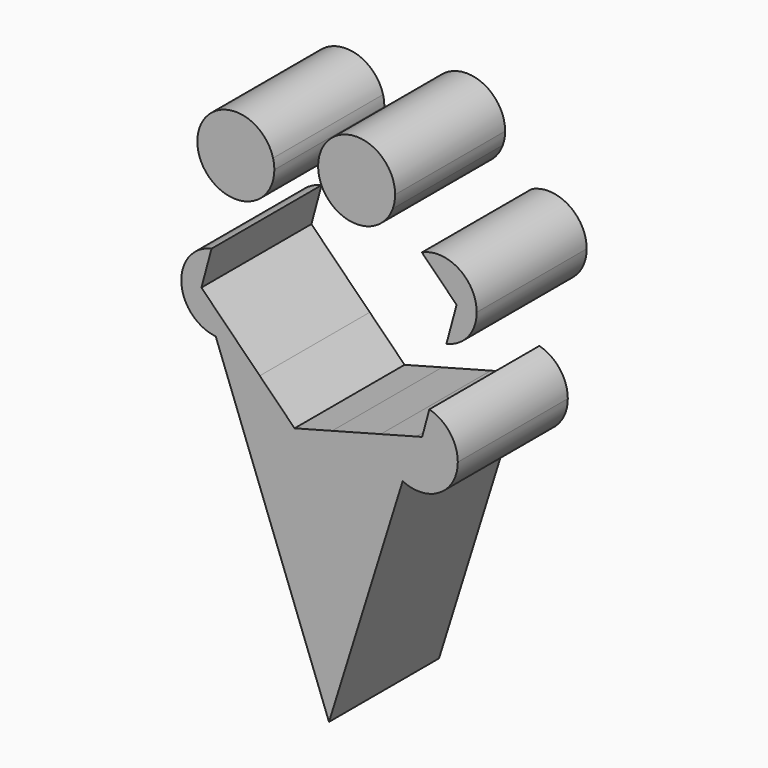
from build123d import *

# Parameters (mm, degrees)
F1_DEPTH = 25


with BuildPart() as f1:
    # F0 (on Front) → F1 (new body)
    with BuildSketch(Plane.XZ):
        with BuildLine():
            Line((18.2441764877, 23.3824430568), (16.9378220156, 18.5476241928))
            Line((16.9378220156, 18.5476241928), (15.8752199276, 18.2652868666))
            Line((15.8752199276, 18.2652868666), (13.3920497807, 10.3127253695))
            ThreePointArc((13.3920497807, 10.3127253695), (20.1476457227, 10.7009431346), (23.4182735487, 16.6247749341))
            ThreePointArc((23.4182735487, 16.6247749341), (21.976210242, 20.8802819207), (18.2441764877, 23.3824430568))
        make_face()
        with BuildLine():
            Line((13.3920497807, 10.3127253695), (15.8752199276, 18.2652868666))
            Line((15.8752199276, 18.2652868666), (9.4186755166, 16.5497590075))
            ThreePointArc((9.4186755166, 16.5497590075), (10.5145101014, 12.8637142914), (13.3920497807, 10.3127253695))
        make_face()
        with BuildLine():
            ThreePointArc((13.3920497807, 10.3127253695), (10.5145101014, 12.8637142914), (9.4186755166, 16.5497590075))
            Line((9.4186755166, 16.5497590075), (0.5681722049, 14.1981473662))
            ThreePointArc((0.5681722049, 14.1981473662), (-8.5434427291, 9.1162877381), (-12.5855881849, 18.734389635))
            Line((-12.5855881849, 18.734389635), (-16.8857592738, 23.0526269106))
            ThreePointArc((-16.8857592738, 23.0526269106), (-18.6970412303, 22.4886563526), (-20.5932388995, 22.4317396104))
            Line((-20.5932388995, 22.4317396104), (0, -32.5764417648))
            Line((0, -32.5764417648), (13.3920497807, 10.3127253695))
        make_face()
        with BuildLine():
            ThreePointArc((-12.5855881849, 18.734389635), (-8.5434427291, 9.1162877381), (0.5681722049, 14.1981473662))
            Line((0.5681722049, 14.1981473662), (-6.2612998485, 12.3835312456))
            Line((-6.2612998485, 12.3835312456), (-12.5855881849, 18.734389635))
        make_face()
        with BuildLine():
            Line((-23.1991218641, 29.3925136519), (-20.5932388995, 22.4317396104))
            ThreePointArc((-20.5932388995, 22.4317396104), (-18.6970412303, 22.4886563526), (-16.8857592738, 23.0526269106))
            Line((-16.8857592738, 23.0526269106), (-23.1991218641, 29.3925136519))
        make_face()
        with BuildLine():
            ThreePointArc((-21.351579017, 36.2302710908), (-26.8426747205, 29.0083871043), (-20.5932388995, 22.4317396104))
            Line((-20.5932388995, 22.4317396104), (-23.1991218641, 29.3925136519))
            Line((-23.1991218641, 29.3925136519), (-21.3515790169, 36.2302710908))
        make_face()
    extrude(amount=F1_DEPTH)


with BuildPart() as f1b:
    # F0 (on Front) → F1, piece 2 (new body)
    with BuildSketch(Plane.XZ):
        with BuildLine():
            Line((23.1991218641, 41.7206995462), (21.3515790169, 34.8829421073))
            ThreePointArc((21.351579017, 34.8829421073), (25.307051013, 37.3325620056), (26.8532221814, 41.7206995462))
            ThreePointArc((26.8532221814, 41.7206995462), (23.6100665785, 47.6271468859), (16.8857592738, 48.0605862875))
            Line((16.8857592738, 48.0605862875), (23.1991218641, 41.7206995462))
        make_face()
    extrude(amount=F1_DEPTH)


with BuildPart() as f1c:
    # F0 (on Front) → F1, piece 3 (new body)
    with BuildSketch(Plane.XZ):
        with BuildLine():
            ThreePointArc((-1.9303688689, 56.5531251129), (3.414311862, 48.916146138), (11.6080114951, 53.3605073181))
            Line((11.6080114951, 53.3605073181), (6.2612998485, 58.7296819525))
            Line((6.2612998485, 58.7296819525), (4.6632730761, 58.3050802966))
            Line((4.6632730761, 58.3050802966), (-1.9303688689, 56.5531251129))
        make_face()
        with BuildLine():
            Line((6.2612998485, 58.7296819525), (11.6080114951, 53.3605073181))
            ThreePointArc((11.6080114951, 53.3605073181), (11.9169654414, 54.5270226619), (12.0209804834, 55.7292670045))
            ThreePointArc((12.0209804834, 55.7292670045), (5.4336271447, 62.7170937577), (-1.9303688689, 56.5531251129))
            Line((-1.9303688689, 56.5531251129), (4.6632730761, 58.3050802966))
            Line((4.6632730761, 58.3050802966), (6.2612998485, 58.7296819525))
        make_face()
    extrude(amount=F1_DEPTH)


with BuildPart() as f1d:
    # F0 (on Front) → F1, piece 4 (new body)
    with BuildSketch(Plane.XZ):
        with BuildLine():
            ThreePointArc((-10.1725582814, 54.3631447367), (-21.8771828108, 57.5257013967), (-18.7637249546, 45.8079208825))
            Line((-18.7637249546, 45.8079208825), (-16.9378220156, 52.5655890053))
            Line((-16.9378220156, 52.5655890053), (-10.1725582814, 54.3631447367))
        make_face()
        with BuildLine():
            Line((-16.9378220156, 52.5655890053), (-18.7637249546, 45.8079208825))
            ThreePointArc((-18.7637249546, 45.8079208825), (-12.6823150289, 47.007652312), (-9.9378220156, 52.5655890053))
            ThreePointArc((-9.9378220156, 52.5655890053), (-9.9967541533, 53.4719978151), (-10.1725582814, 54.3631447367))
            Line((-10.1725582814, 54.3631447367), (-16.9378220156, 52.5655890053))
        make_face()
    extrude(amount=F1_DEPTH)


solid = Compound([f1.part, f1b.part, f1c.part, f1d.part])
